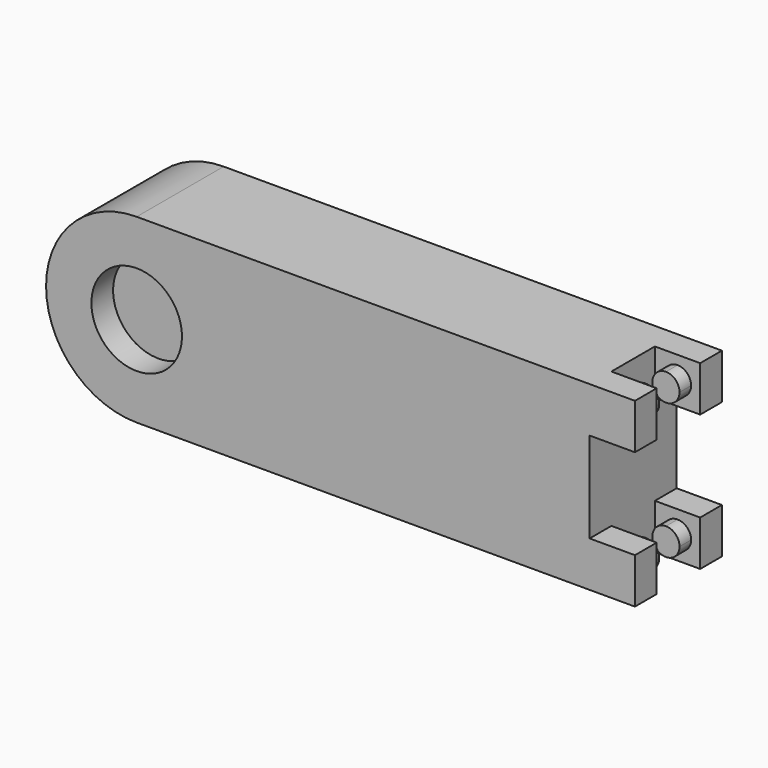
from build123d import *
from build123d import SkipClean  # not in build123d's __all__

# Parameters (mm, degrees)
F0_R      = 6.35
F1_DEPTH  = 25.4
F2_R      = 6.35
F3_DEPTH  = 25.4
F4_DEPTH  = 5.08
F5_DEPTH  = 8.89
F6_DEPTH  = 20.32
F7_DEPTH  = 10.16
F8_DEPTH  = 5.08
F9_DEPTH  = 13.97
F10_DEPTH = 3.81
F11_W     = 3.81
F11_H     = 6.35
F12_DEPTH = 6.35
F17_DEPTH = 2.032
F18_DEPTH = 2.032


with BuildPart() as f1:
    # F0 (on Front) → F1 (new body)
    with BuildSketch(Plane.XZ):
        with BuildLine():
            ThreePointArc((42.0866659097, -2.2684633732), (38.3669220307, 6.7117927479), (29.3866659097, 10.4315366268))
            ThreePointArc((29.3866659097, 10.4315366268), (20.4064097886, 6.7117927479), (16.6866659097, -2.2684633732))
            ThreePointArc((16.6866659097, -2.2684633732), (20.4064097886, -11.2487194943), (29.3866659097, -14.9684633732))
            ThreePointArc((29.3866659097, -14.9684633732), (38.3669220307, -11.2487194943), (42.0866659097, -2.2684633732))
        make_face()
        with Locations((29.3866659097, -2.2684633732)):
            Circle(F0_R, mode=Mode.SUBTRACT)
        with Locations((29.3866659097, -2.2684633732)):
            Circle(F0_R)
        with BuildLine():
            Line((92.8866659097, 10.4315366268), (29.3866659097, 10.4315366268))
            ThreePointArc((29.3866659097, 10.4315366268), (38.3669220307, 6.7117927479), (42.0866659097, -2.2684633732))
            ThreePointArc((42.0866659097, -2.2684633732), (38.3669220307, -11.2487194943), (29.3866659097, -14.9684633732))
            Line((29.3866659097, -14.9684633732), (92.8866659097, -14.9684633732))
            Line((92.8866659097, -14.9684633732), (92.8866659097, 10.4315366268))
        make_face()
    extrude(amount=-F1_DEPTH)

    # F2 (on face) → F3 (cut, through all)
    with BuildSketch(Plane(origin=(0, 25.4, 0), x_dir=(-1, 0, 0), z_dir=(0, 1, 0))):
        with BuildLine():
            ThreePointArc((-29.3866659097, -14.9684633732), (-42.0866659097, -2.2684633732), (-29.3866659097, 10.4315366268))
            Line((-29.3866659097, 10.4315366268), (-92.8866659097, 10.4315366268))
            Line((-92.8866659097, 10.4315366268), (-92.8866659097, -14.9684633732))
            Line((-92.8866659097, -14.9684633732), (-29.3866659097, -14.9684633732))
        make_face()
        with Locations((-29.3866659097, -2.2684633732)):
            Circle(F2_R)
    with SkipClean():  # cleaning this boolean's faces spoils the solid; the shape is the same uncleaned
        extrude(amount=-F3_DEPTH, mode=Mode.SUBTRACT)

    # F2 (on face) → F4 (join)
    with BuildSketch(Plane(origin=(0, 25.4, 0), x_dir=(-1, 0, 0), z_dir=(0, 1, 0))):
        with BuildLine():
            ThreePointArc((-29.3866659097, -14.9684633732), (-42.0866659097, -2.2684633732), (-29.3866659097, 10.4315366268))
            Line((-29.3866659097, 10.4315366268), (-92.8866659097, 10.4315366268))
            Line((-92.8866659097, 10.4315366268), (-92.8866659097, -14.9684633732))
            Line((-92.8866659097, -14.9684633732), (-29.3866659097, -14.9684633732))
        make_face()
    extrude(amount=-F4_DEPTH)

    # F2 (on face) → F5 (join)
    with BuildSketch(Plane(origin=(0, 25.4, 0), x_dir=(-1, 0, 0), z_dir=(0, 1, 0))):
        with Locations((-29.3866659097, -2.2684633732)):
            Circle(F2_R)
    extrude(amount=-F5_DEPTH)

    # F2 (on face) → F6 (join)
    with BuildSketch(Plane(origin=(0, 25.4, 0), x_dir=(-1, 0, 0), z_dir=(0, 1, 0))):
        with BuildLine():
            ThreePointArc((-29.3866659097, -14.9684633732), (-42.0866659097, -2.2684633732), (-29.3866659097, 10.4315366268))
            Line((-29.3866659097, 10.4315366268), (-92.8866659097, 10.4315366268))
            Line((-92.8866659097, 10.4315366268), (-92.8866659097, -14.9684633732))
            Line((-92.8866659097, -14.9684633732), (-29.3866659097, -14.9684633732))
        make_face()
        with Locations((-29.3866659097, -2.2684633732)):
            Circle(F2_R)
    extrude(amount=-F6_DEPTH)

    # F7 (cut): a face of the model
    f7_faces = [f1.faces().sort_by_distance(p)[0] for p in [
        (29.3866659097, 0, 10.072326382),
    ]]
    extrude(f7_faces, amount=-F7_DEPTH, mode=Mode.SUBTRACT)

    # F8 (cut): a face of the model
    f8_faces = [f1.faces().sort_by_distance(p)[0] for p in [
        (66.0488875518, 5.08, -2.2684633732),
    ]]
    extrude(f8_faces, amount=-F8_DEPTH, mode=Mode.SUBTRACT)

    # F0 (on Front) → F9 (cut)
    with BuildSketch(Plane.XZ):
        with Locations((29.3866659097, -2.2684633732)):
            Circle(F0_R)
    extrude(amount=-F9_DEPTH, mode=Mode.SUBTRACT)

    # F2 (on face) → F10 (cut)
    with BuildSketch(Plane(origin=(0, 25.4, 0), x_dir=(-1, 0, 0), z_dir=(0, 1, 0))):
        with Locations((-29.3866659097, -2.2684633732)):
            Circle(F2_R)
    extrude(amount=-F10_DEPTH, mode=Mode.SUBTRACT)

    # F11 (on face) → F12 (join)
    with BuildSketch(Plane.YZ.offset(92.8866659097)):
        with Locations((12.065, 7.2565366268)):
            Rectangle(F11_W, F11_H)
        with Locations((23.495, 7.2565366268)):
            Rectangle(F11_W, F11_H)
        with Locations((23.495, -11.7934633732)):
            Rectangle(F11_W, F11_H)
        with Locations((12.065, -11.7934633732)):
            Rectangle(F11_W, F11_H)
    extrude(amount=F12_DEPTH)

    # F15 (on face) + F13 (on face) → F17 (join)
    with BuildSketch(Plane(origin=(0, 13.97, 0), x_dir=(-1, 0, 0), z_dir=(0, 1, 0))):
        with BuildLine():
            Line((-96.0616659097, -11.7934633732), (-94.1566659097, -11.7934633732))
            ThreePointArc((-94.1566659097, -11.7934633732), (-94.7146274915, -10.446424955), (-96.0616659097, -9.8884633732))
            Line((-96.0616659097, -9.8884633732), (-96.0616659097, -11.7934633732))
        make_face()
        with BuildLine():
            Line((-97.9666659097, -11.7934633732), (-96.0616659097, -11.7934633732))
            Line((-96.0616659097, -11.7934633732), (-96.0616659097, -9.8884633732))
            ThreePointArc((-96.0616659097, -9.8884633732), (-97.4087043278, -10.446424955), (-97.9666659097, -11.7934633732))
        make_face()
        with BuildLine():
            Line((-96.0616659097, -13.6984633732), (-96.0616659097, -11.7934633732))
            Line((-96.0616659097, -11.7934633732), (-97.9666659097, -11.7934633732))
            ThreePointArc((-97.9666659097, -11.7934633732), (-97.4087043278, -13.1405017913), (-96.0616659097, -13.6984633732))
        make_face()
        with BuildLine():
            ThreePointArc((-96.0616659097, -13.6984633732), (-94.7146274915, -13.1405017913), (-94.1566659097, -11.7934633732))
            Line((-94.1566659097, -11.7934633732), (-96.0616659097, -11.7934633732))
            Line((-96.0616659097, -11.7934633732), (-96.0616659097, -13.6984633732))
        make_face()
    with BuildSketch(Plane(origin=(0, 13.97, 0), x_dir=(-1, 0, 0), z_dir=(0, 1, 0))):
        with BuildLine():
            Line((-96.0616659097, 7.2565366268), (-96.0616659097, 9.1615366268))
            ThreePointArc((-96.0616659097, 9.1615366268), (-97.4087043278, 8.603575045), (-97.9666659097, 7.2565366268))
            Line((-97.9666659097, 7.2565366268), (-96.0616659097, 7.2565366268))
        make_face()
        with BuildLine():
            Line((-96.0616659097, 7.2565366268), (-94.1566659097, 7.2565366268))
            ThreePointArc((-94.1566659097, 7.2565366268), (-94.7146274915, 8.603575045), (-96.0616659097, 9.1615366268))
            Line((-96.0616659097, 9.1615366268), (-96.0616659097, 7.2565366268))
        make_face()
        with BuildLine():
            ThreePointArc((-97.9666659097, 7.2565366268), (-97.4087043278, 5.9094982087), (-96.0616659097, 5.3515366268))
            Line((-96.0616659097, 5.3515366268), (-96.0616659097, 7.2565366268))
            Line((-96.0616659097, 7.2565366268), (-97.9666659097, 7.2565366268))
        make_face()
        with BuildLine():
            ThreePointArc((-96.0616659097, 5.3515366268), (-94.7146274915, 5.9094982087), (-94.1566659097, 7.2565366268))
            Line((-94.1566659097, 7.2565366268), (-96.0616659097, 7.2565366268))
            Line((-96.0616659097, 7.2565366268), (-96.0616659097, 5.3515366268))
        make_face()
    extrude(amount=F17_DEPTH)

    # F14 (on face) + F16 (on face) → F18 (join)
    with BuildSketch(Plane.XZ.offset(-21.59)):
        with BuildLine():
            Line((96.0616659097, 7.2565366268), (96.0616659097, 9.1615366268))
            ThreePointArc((96.0616659097, 9.1615366268), (94.7146274915, 8.603575045), (94.1566659097, 7.2565366268))
            Line((94.1566659097, 7.2565366268), (96.0616659097, 7.2565366268))
        make_face()
        with BuildLine():
            Line((96.0616659097, 7.2565366268), (97.9666659097, 7.2565366268))
            ThreePointArc((97.9666659097, 7.2565366268), (97.4087043278, 8.603575045), (96.0616659097, 9.1615366268))
            Line((96.0616659097, 9.1615366268), (96.0616659097, 7.2565366268))
        make_face()
        with BuildLine():
            ThreePointArc((96.0616659097, 5.3515366268), (97.4087043278, 5.9094982087), (97.9666659097, 7.2565366268))
            Line((97.9666659097, 7.2565366268), (96.0616659097, 7.2565366268))
            Line((96.0616659097, 7.2565366268), (96.0616659097, 5.3515366268))
        make_face()
        with BuildLine():
            ThreePointArc((94.1566659097, 7.2565366268), (94.7146274915, 5.9094982087), (96.0616659097, 5.3515366268))
            Line((96.0616659097, 5.3515366268), (96.0616659097, 7.2565366268))
            Line((96.0616659097, 7.2565366268), (94.1566659097, 7.2565366268))
        make_face()
    with BuildSketch(Plane.XZ.offset(-21.59)):
        with BuildLine():
            Line((94.1566659097, -11.7934633732), (96.0616659097, -11.7934633732))
            Line((96.0616659097, -11.7934633732), (96.0616659097, -9.8884633732))
            ThreePointArc((96.0616659097, -9.8884633732), (94.7146274915, -10.446424955), (94.1566659097, -11.7934633732))
        make_face()
        with BuildLine():
            Line((96.0616659097, -9.8884633732), (96.0616659097, -11.7934633732))
            Line((96.0616659097, -11.7934633732), (97.9666659097, -11.7934633732))
            ThreePointArc((97.9666659097, -11.7934633732), (97.4087043278, -10.446424955), (96.0616659097, -9.8884633732))
        make_face()
        with BuildLine():
            Line((96.0616659097, -11.7934633732), (96.0616659097, -13.6984633732))
            ThreePointArc((96.0616659097, -13.6984633732), (97.4087043278, -13.1405017913), (97.9666659097, -11.7934633732))
            Line((97.9666659097, -11.7934633732), (96.0616659097, -11.7934633732))
        make_face()
        with BuildLine():
            ThreePointArc((94.1566659097, -11.7934633732), (94.7146274915, -13.1405017913), (96.0616659097, -13.6984633732))
            Line((96.0616659097, -13.6984633732), (96.0616659097, -11.7934633732))
            Line((96.0616659097, -11.7934633732), (94.1566659097, -11.7934633732))
        make_face()
    extrude(amount=F18_DEPTH)


solid = f1.part
